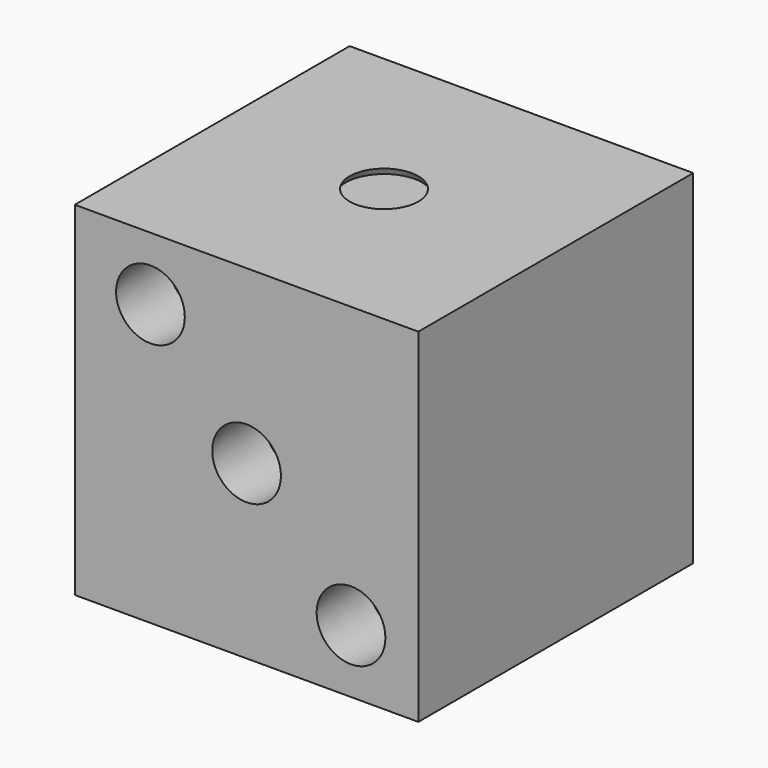
from build123d import *

# Parameters (mm, degrees)
F0_W     = 25.4
F0_H     = 25.4
F1_DEPTH = 25.4
F2_R     = 2.54
F3_DEPTH = 0.508
F3_TAPER = -30
F4_R     = 2.54
F5_DEPTH = 5.08
F5_TAPER = -3


# Not quite as in the source:
# - the program builds the solid bodies; features that only make, move or delete a surface that nothing else refers to are left out


with BuildPart() as f1:
    # F0 (on Front) → F1 (new body)
    with BuildSketch(Plane.XZ):
        Rectangle(F0_W, F0_H)
    extrude(amount=F1_DEPTH)

    # F2 (on face) → F3 (cut)
    with BuildSketch(Plane.XY.offset(12.7)):
        with Locations((0, -12.7)):
            Circle(F2_R)
    extrude(amount=-F3_DEPTH, taper=F3_TAPER, mode=Mode.SUBTRACT)

    # F4 (on face) → F5 (cut)
    with BuildSketch(Plane.XZ.offset(25.4)):
        Circle(F4_R)
        with Locations((-7.1051362902, 8.0318916589)):
            Circle(F4_R)
        with Locations((7.7229747549, -8.0318916589)):
            Circle(F4_R)
    extrude(amount=-F5_DEPTH, taper=F5_TAPER, mode=Mode.SUBTRACT)


solid = f1.part
